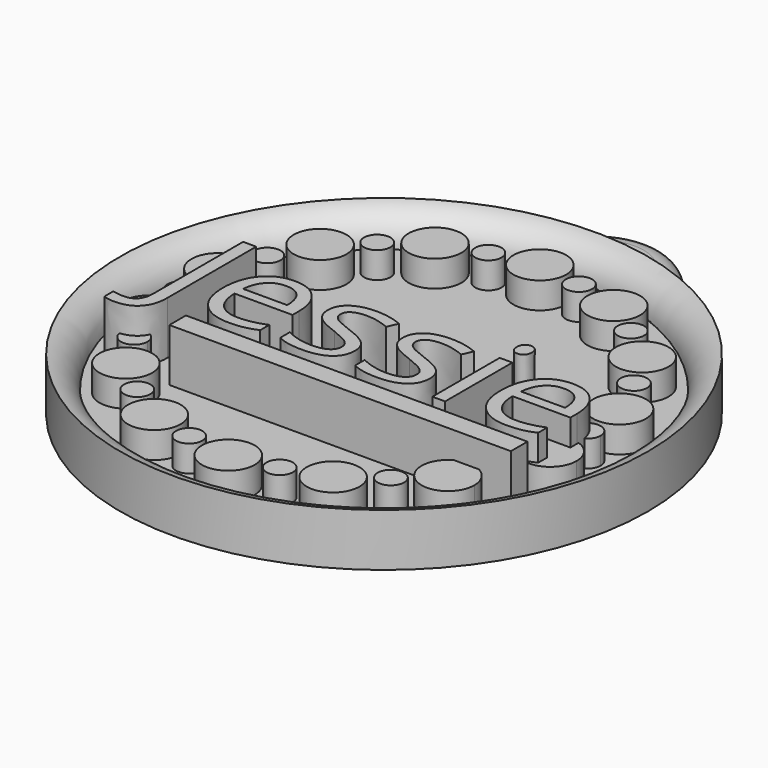
from build123d import *

# Parameters (mm, degrees)
F0_R         = 22.5
F1_DEPTH     = 2
F0_R_2       = 25
F2_DEPTH     = 5
F3_TEXT_SIZE = 14.8871830658
F4_DEPTH     = 5
F6_W         = 32.35121537
F6_H         = 1.9594812766
F7_DEPTH     = 5
F8_R         = 2.5
F9_DEPTH     = 2.5
F10_R        = 1.25
F11_DEPTH    = 2.5
F13_DEPTH    = 2
F14_R        = 1.99999
F15_R        = 1.8080611008
F16_DEPTH    = 2


# Not quite as in the source:
# - a fillet or chamfer that OpenCascade refuses, or shapes differently, is made with other operations: its cross-section is extruded or revolved along the edge and cut away or added
# - a fillet or chamfer is up to 0.001 mm smaller than in the source, because OpenCascade refuses the exact size
# - Text() gives the source's letters only with a copy of the font that has no kerning and outlines rounded to 1/6400 em; it was checked with that copy


with BuildPart() as f1:
    # F0 (on Top) → F1 (new body)
    with BuildSketch(Plane.XY):
        Circle(F0_R)
    extrude(amount=F1_DEPTH)

    # F0 (on Top) → F2 (join)
    with BuildSketch(Plane.XY):
        Circle(F0_R_2)
        Circle(F0_R, mode=Mode.SUBTRACT)
    extrude(amount=F2_DEPTH)

    # F3 (on face) → F4 (join)
    with BuildSketch(Plane.XY.offset(2)):
        with Locations((-18.3453189751, -6.1094017471)):
            Text('Jessie', F3_TEXT_SIZE, font='Open Sans', text_align=(TextAlign.LEFT, TextAlign.BOTTOM))
    extrude(amount=F4_DEPTH)

    # F5: fillet of radius 3 on 1 edges, made by hand

    # F5_s1 → F5_t2 (revolve, cut)
    with BuildSketch(Plane.XZ):
        with BuildLine():
            ThreePointArc((25, 5), (23.2087121525, 3.9784517816), (22.5, 2.0419601084))
            Line((22.5, 2.0419601084), (22.5, 5))
            Line((22.5, 5), (25, 5))
        make_face()
    revolve(axis=Axis((0, 0, 5), (0, 0, 1)), mode=Mode.SUBTRACT)

    # F6 (on face) → F7 (join)
    with BuildSketch(Plane.XY.offset(2)):
        with Locations((3.2768319361, -8.3178333007)):
            Rectangle(F6_W, F6_H)
    extrude(amount=F7_DEPTH)

    # F8 (on face) → F9 (join)
    with BuildSketch(Plane.XY.offset(2)):
        with Locations((-8.755111918, 16.978919224)):
            Circle(F8_R)
        with Locations((-0.5212063777, 19.096178325)):
            Circle(F8_R)
        with Locations((7.815930539, 17.4312051368)):
            Circle(F8_R)
        with Locations((14.6050265545, 12.3137679876)):
            Circle(F8_R)
        with Locations((18.5014179388, 4.7574380672)):
            Circle(F8_R)
        with BuildLine():
            ThreePointArc((17.9969326039, -6.1302297189), (20.2181139471, -5.752517313), (21.2333765912, -3.7411608095))
            ThreePointArc((21.2333765912, -3.7411608095), (20.7610171183, -2.27874025), (19.522437477, -1.3689502542))
            add(Edge.make_bspline(
                [(19.526279071, -1.5804415238), (19.526279071, -1.4733103541), (19.522437477, -1.3689502542)],
                knots=[0, 0, 0, 0.0663626655, 0.0663626655, 0.0663626655], degree=2))
            Line((19.526279071, -1.5804415238), (19.526279071, -2.343409656))
            Line((19.526279071, -2.343409656), (16.6606267962, -2.343409656))
            ThreePointArc((16.6606267962, -2.343409656), (16.2336498563, -3.7781236371), (16.7028603529, -5.199585921))
            add(Edge.make_bspline(
                [(19.184339085, -4.6625536429), (17.958011131, -5.1871494899), (16.7028603529, -5.199585921)],
                knots=[0, 0, 0, 0.97629331, 0.97629331, 0.97629331], degree=2))
            Line((19.184339085, -4.6625536429), (19.184339085, -5.7395482929))
            add(Edge.make_bspline(
                [(17.9969326039, -6.1302297189), (18.5570870019, -6.0086964594), (19.184339085, -5.7395482929)],
                knots=[6.7531569629, 6.7531569629, 6.7531569629, 7.2281974814, 7.2281974814, 7.2281974814], degree=2))
        make_face()
        with BuildLine():
            ThreePointArc((14.0697575291, -9.297573939), (13.9729709455, -13.6450535431), (17.7549602557, -11.4987769048))
            ThreePointArc((17.7549602557, -11.4987769048), (17.4012368941, -10.2167875945), (16.4401629824, -9.297573939))
            Line((16.4401629824, -9.297573939), (14.0697575291, -9.297573939))
        make_face()
        with Locations((8.7551119484, -16.9789192083)):
            Circle(F8_R)
        with Locations((0.5212063434, -19.096178326)):
            Circle(F8_R)
        with Locations((-7.8159305703, -17.4312051227)):
            Circle(F8_R)
        with Locations((-14.6050265766, -12.3137679614)):
            Circle(F8_R)
        with BuildLine():
            Line((-16.9636022968, -6.1094017471), (-16.9636022968, -2.7863664918))
            ThreePointArc((-16.9636022968, -2.7863664918), (-21.0009094778, -4.7070188995), (-17.0443408684, -6.7889218233))
            add(Edge.make_bspline(
                [(-16.9636022968, -6.1094017471), (-16.9636022968, -6.4906594051), (-17.0443408684, -6.7889218233)],
                knots=[0, 0, 0, 0.4643135047, 0.4643135047, 0.4643135047], degree=2))
        make_face()
        with BuildLine():
            ThreePointArc((-16.357348679, 4.5186512884), (-21.1652372457, 4.3208622526), (-16.9636022968, 1.9754035069))
            Line((-16.9636022968, 1.9754035069), (-16.9636022968, 4.5186512884))
            Line((-16.9636022968, 4.5186512884), (-16.357348679, 4.5186512884))
        make_face()
        with Locations((-15.2549602351, 11.4987769322)):
            Circle(F8_R)
    extrude(amount=F9_DEPTH)

    # F10 (on face) → F11 (join)
    with BuildSketch(Plane.XY.offset(2)):
        with Locations((-12.1662989259, 14.3955266103)):
            Circle(F10_R)
        with Locations((-17.2074414821, 7.6911620438)):
            Circle(F10_R)
        with Locations((-18.8404392173, -0.5365314914)):
            Circle(F10_R)
        with BuildLine():
            ThreePointArc((-17.9716308535, -8.8819138042), (-16.6294234524, -9.9028916035), (-15.4918569027, -8.6579583847))
            ThreePointArc((-15.4918569027, -8.6579583847), (-15.6423946991, -8.0632459644), (-16.0577494832, -7.6117762597))
            add(Edge.make_bspline(
                [(-17.9716308535, -8.8819138042), (-16.9954528066, -8.7677107524), (-16.2078166598, -7.9105000794), (-16.0577494832, -7.6117762597)],
                knots=[1.3542446333, 1.3542446333, 1.3542446333, 2.9215017065, 3.5230101719, 3.5230101719, 3.5230101719], degree=2))
        make_face()
        with BuildLine():
            add(Edge.make_bspline(
                [(-17.9716308535, -8.8819138042), (-16.9954528066, -8.7677107524), (-16.2078166598, -7.9105000794), (-16.0577494832, -7.6117762597)],
                knots=[1.3542446333, 1.3542446333, 1.3542446333, 2.9215017065, 3.5230101719, 3.5230101719, 3.5230101719], degree=2))
            ThreePointArc((-16.0577494832, -7.6117762597), (-17.433051764, -7.6164452241), (-17.9716308535, -8.8819138042))
        make_face()
        with Locations((-11.3273445032, -15.0645704369)):
            Circle(F10_R)
        with Locations((-3.669312604, -18.4874595593)):
            Circle(F10_R)
        with Locations((4.7154716576, -18.2486805821)):
            Circle(F10_R)
        with Locations((12.1662989259, -14.3955266103)):
            Circle(F10_R)
        with BuildLine():
            Line((16.0083409809, -7.3380926624), (18.4065419832, -7.3380926624))
            ThreePointArc((18.4065419832, -7.3380926624), (17.2074414821, -6.4411620438), (16.0083409809, -7.3380926624))
        make_face()
        with BuildLine():
            ThreePointArc((19.4278430246, -0.5668527422), (19.912062929, -0.106992106), (20.0904392173, 0.5365314914))
            ThreePointArc((20.0904392173, 0.5365314914), (19.3892908317, 1.6595906641), (18.0724201688, 1.5227600355))
            add(Edge.make_bspline(
                [(19.4278430246, -0.5668527422), (19.2332511577, 0.3648135799), (18.3914385199, 1.3155006522), (18.0724201688, 1.5227600355)],
                knots=[0.3359271998, 0.3359271998, 0.3359271998, 1, 1.3009812078, 1.3009812078, 1.3009812078], degree=2))
        make_face()
        with BuildLine():
            add(Edge.make_bspline(
                [(19.4278430246, -0.5668527422), (19.2332511577, 0.3648135799), (18.3914385199, 1.3155006522), (18.0724201688, 1.5227600355)],
                knots=[0.3359271998, 0.3359271998, 0.3359271998, 1, 1.3009812078, 1.3009812078, 1.3009812078], degree=2))
            ThreePointArc((18.0724201688, 1.5227600355), (17.7917372308, -0.1437068076), (19.4278430246, -0.5668527422))
        make_face()
        with Locations((16.7418569027, 8.6579583847)):
            Circle(F10_R)
        with Locations((11.3273445032, 15.0645704369)):
            Circle(F10_R)
        with Locations((3.669312604, 18.4874595593)):
            Circle(F10_R)
        with Locations((-4.7154716576, 18.2486805821)):
            Circle(F10_R)
    extrude(amount=F11_DEPTH)

    # F12 (on face) → F13 (join)
    with BuildSketch(Plane.XY):
        with BuildLine():
            ThreePointArc((6.4348667538, 24.1576590311), (6.4859004584, 24.6256642499), (6.502941464, 25.096135214))
            ThreePointArc((6.502941464, 25.096135214), (-0.4704709641, 31.5820356724), (-6.4348667538, 24.1576590311))
            ThreePointArc((-6.4348667538, 24.1576590311), (0, 25), (6.4348667538, 24.1576590311))
        make_face()
        with BuildLine():
            ThreePointArc((6.4348667538, 24.1576590311), (0, 25), (-6.4348667538, 24.1576590311))
            ThreePointArc((-6.4348667538, 24.1576590311), (-6.1330164739, 22.9341091697), (-5.6008331154, 21.7917568914))
            ThreePointArc((-5.6008331154, 21.7917568914), (0, 22.5), (5.6008331154, 21.7917568914))
            ThreePointArc((5.6008331154, 21.7917568914), (6.1330164739, 22.9341091697), (6.4348667538, 24.1576590311))
        make_face()
    extrude(amount=F13_DEPTH)

    # F14 (radius 2 in the source; OpenCascade refuses exactly that, so slightly less here)
    f14_edges = [f1.edges().sort_by_distance(p)[0] for p in [
        (0, 31.599077, 2),
    ]]
    fillet(f14_edges, radius=F14_R)

    # F15 (on face) → F16 (cut)
    with BuildSketch(Plane.XY.offset(2)):
        with Locations((0, 27.0812753588)):
            Circle(F15_R)
    extrude(amount=-F16_DEPTH, mode=Mode.SUBTRACT)


solid = f1.part
